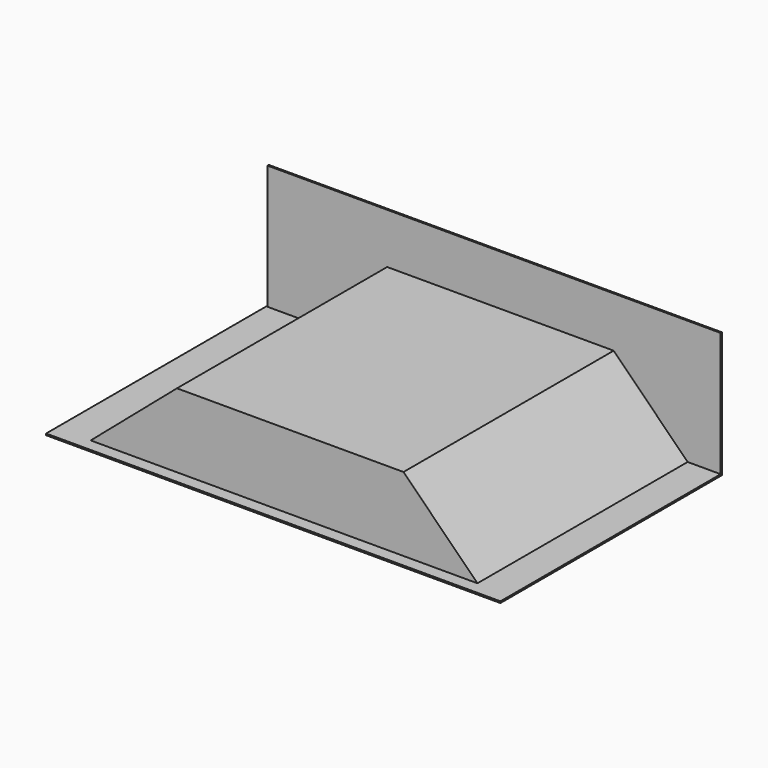
from build123d import *

# Parameters (mm, degrees)
F1_DEPTH    = 3.175
F2_START    = 3.048
F2_DEPTH    = 530.352
F3_T        = 2.54
F3_T3_DEPTH = 8.128
F3_T5_DEPTH = 220.6061469057
F3_T7_DEPTH = 239.2564292152
F3_T9_DEPTH = 462.28
F5_DEPTH    = 3.175


# Not quite as in the source:
# - a shell that OpenCascade refuses in one call is made with other operations: the cavity is built on its own and cut out


with BuildPart() as f1:
    # F0 (on Front) → F1 (new body)
    with BuildSketch(Plane.XZ):
        Polygon((-63.5, 0), (0, 0), (0, 254), (-914.4, 254), (-914.4, 0), (-850.9, 0), (-673.1, 152.4), (-215.9, 152.4), align=None)
    extrude(amount=F1_DEPTH)

    # F0 (on Front) → F2 (join)
    with BuildSketch(Plane.XZ.offset(F2_START)):
        Polygon((-850.9, 0), (-63.5, 0), (-215.9, 152.4), (-673.1, 152.4), align=None)
    extrude(amount=F2_DEPTH)

    # F3: shell of thickness 2.54, made by hand


with BuildPart() as f3_core1:
    # F3_t2: copy of F1
    add(f1.part)

    # the walls: a layer under each face that stays
    f3_faces = [f3_core1.faces().sort_by_distance(p)[0] for p in [
        (-139.7, -1.524, 76.2),
        (-762, 0, 127),
        (-444.5, -1.524, 152.4),
        (0, -1.5875, 127),
        (-457.2, -1.5875, 254),
        (-914.4, -1.5875, 127),
        (-762, -1.524, 76.2),
        (-762, -3.175, 127),
        (-762, -268.2875, 76.2),
        (-139.7, -268.2875, 76.2),
        (-457.2, -533.4, 76.2),
        (-444.5, -268.2875, 152.4),
    ]]
    thicken(f3_faces, amount=-F3_T, mode=Mode.SUBTRACT)

    # F3_s4 → F3_t3 (cut)
    with BuildSketch(Plane.XZ.offset(-2.54)):
        Polygon((-215.9179605122, 152.3566394878), (-214.1039487758, 154.1960512242), (-214.8478975516, 154.94), (-215.9, 154.94), align=None)
        Polygon((-673.0834698991, 152.3553148823), (-673.1, 154.94), (-674.0396071536, 154.94), (-674.7530100886, 154.32851177), align=None)
    extrude(amount=F3_T3_DEPTH, mode=Mode.SUBTRACT)

    # F3_s6 → F3_t5 (cut)
    with BuildSketch(Plane(origin=(-185.9460512242, 0, 185.9460512242), x_dir=(0, 1, 0), z_dir=(0.7071067812, 0, -0.7071067812))):
        Polygon((-3.2004, -44.8758806053), (-0.635, -44.9012806053), (-0.635, -47.4412806053), (-3.175, -47.4412806053), align=None)
    extrude(amount=F3_T5_DEPTH, mode=Mode.SUBTRACT)

    # F3_s8 → F3_t7 (cut)
    with BuildSketch(Plane(origin=(-492.4473352994, 0, -422.0977159709), x_dir=(0, 1, 0), z_dir=(0.7592566024, 0, 0.6507913735))):
        Polygon((-3.2004, 553.7837796737), (-0.635, 553.7583796737), (-0.635, 551.2183796737), (-3.175, 551.2183796737), align=None)
    extrude(amount=F3_T7_DEPTH, mode=Mode.SUBTRACT)

    # F3_s10 → F3_t9 (cut)
    with BuildSketch(Plane.YZ.offset(-675.64)):
        Polygon((-3.2004, 152.4254), (-0.635, 152.4), (-0.635, 149.86), (-3.175, 149.86), align=None)
    extrude(amount=F3_T9_DEPTH, mode=Mode.SUBTRACT)


with BuildPart() as f1_1:
    add(f1.part)

    # what is left inside the walls is the cavity
    f3_cavity = [f3_core1.part.solids().sort_by_distance(p)[0] for p in [
        (-457.044581, -354.922667, 0.0254),
    ]]
    add(f3_cavity, mode=Mode.SUBTRACT)

    # F4 (on Top) → F5 (join)
    with BuildSketch(Plane.XY):
        Polygon((0, -558.8), (0, 0), (-69.1089183092, 0), (-69.1089183092, -530.9250950813), (-844.7285890579, -530.9250950813), (-844.7285890579, 0), (-916.9259883143, 0), (-916.9259883143, -558.8), align=None)
    extrude(amount=F5_DEPTH)


solid = f1_1.part
